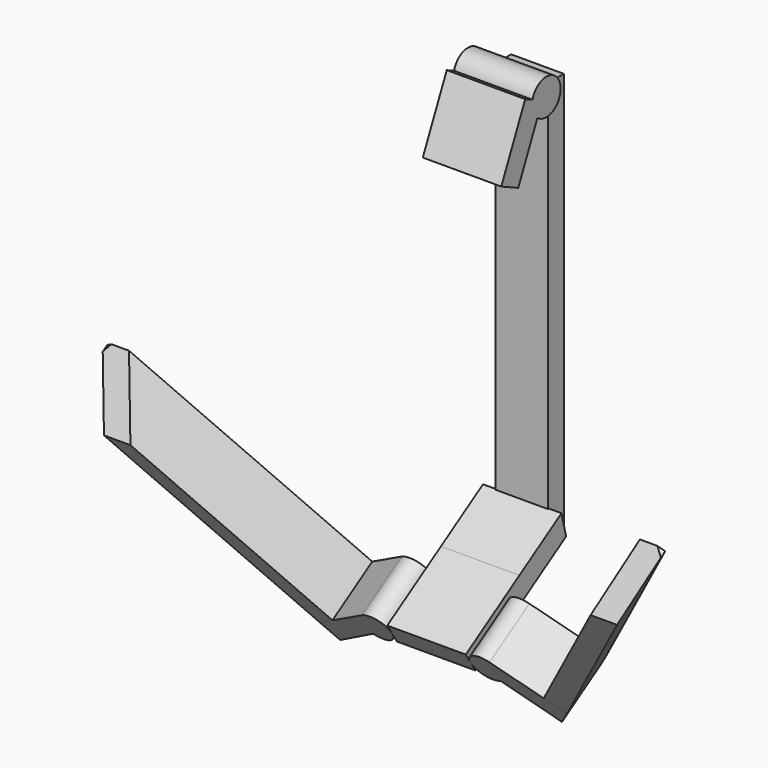
from build123d import *

# Parameters (mm, degrees)
F0_W           = 34.1221652925
F0_H           = 261.6441845894
F1_DEPTH       = 12.7
F3_DEPTH       = 25.4
F3_DEPTH_BACK  = 25.4
F7_DEPTH       = 25.4
F7_DEPTH_BACK  = 25.4
F9_DEPTH       = 38.1
F11_W          = 14.1206162959
F11_H          = 38.1
F12_DEPTH      = 177.8
F15_DEPTH      = 508
F15_DEPTH_BACK = 508
F20_DEPTH      = 228.6
F20_DEPTH_BACK = 228.6


with BuildPart() as f1:
    # F0 (on Front) → F1 (new body)
    with BuildSketch(Plane.XZ):
        Rectangle(F0_W, F0_H)
    extrude(amount=F1_DEPTH)


with BuildPart() as f3:
    # F2 (on Right) → F3 (new body, two sides)
    with BuildSketch(Plane.YZ) as f3_sk:
        with BuildLine():
            ThreePointArc((-31.7653294782, 121.3009119591), (-19.5443195923, 119.9093799667), (-12.9962554201, 130.3215026855))
            ThreePointArc((-12.9962554201, 130.3215026855), (-23.058684097, 141.777262991), (-35.7164542609, 133.2762177888))
            ThreePointArc((-35.7164542609, 133.2762177888), (-35.5190055596, 126.7018951749), (-31.7653294782, 121.3009119591))
        make_face()
        with BuildLine():
            ThreePointArc((-31.7653294782, 121.3009119591), (-35.5190055596, 126.7018951749), (-35.7164542609, 133.2762177888))
            Line((-35.7164542609, 133.2762177888), (-41.654221951, 136.0218451646))
            Line((-41.654221951, 136.0218451646), (-61.046799285, 94.0829352683))
            Line((-61.046799285, 94.0829352683), (-47.2919270396, 87.7226740122))
            Line((-47.2919270396, 87.7226740122), (-31.7653294782, 121.3009119591))
        make_face()
    extrude(amount=F3_DEPTH)
    extrude(f3_sk.sketch, amount=-F3_DEPTH_BACK)


with BuildPart() as f4_1:
    # F4: instance of F3
    add(f3.part.mirror(Plane.XY))


with BuildPart() as f7:
    # F6 (on Right) → F7 (new body, two sides)
    with BuildSketch(Plane.YZ) as f7_sk:
        Polygon((-82.0237547159, -173.1977909803), (-37.7950449612, -145.1887713173), (-8.5108920135, -126.643794078), (-12.3146369824, -111.9083875607), (-46.3577486399, -133.4671033607), (-89.7730322343, -160.9609990365), align=None)
    extrude(amount=F7_DEPTH)
    extrude(f7_sk.sketch, amount=-F7_DEPTH_BACK)


with BuildPart() as f9:
    # F8 (on face) → F9 (new body)
    with BuildSketch(Plane(origin=(0, -136.8311862758, -86.652027793), x_dir=(1, 0, 0), z_dir=(0, -0.8448406307, -0.5350180453))):
        with BuildLine():
            ThreePointArc((-41.2132547892, -103.603452681), (-30.7810506283, -104.152405518), (-25.4, -95.198270886))
            ThreePointArc((-25.4, -95.198270886), (-30.8167276914, -86.225263874), (-41.2799833491, -86.8385132228))
            ThreePointArc((-41.2799833491, -86.8385132228), (-45.680760801, -95.2386319206), (-41.2132547892, -103.603452681))
        make_face()
        with BuildLine():
            ThreePointArc((-41.2132547892, -103.603452681), (-45.680760801, -95.2386319206), (-41.2799833491, -86.8385132228))
            Line((-41.2799833491, -86.8385132228), (-80.0200754217, -113.4363166259))
            Line((-80.0200754217, -113.4363166259), (-71.7834234238, -125.1321434975))
            Line((-71.7834234238, -125.1321434975), (-41.2132547892, -103.603452681))
        make_face()
    extrude(amount=-F9_DEPTH)


with BuildPart() as f10_1:
    # F10: instance of F9
    add(f9.part.mirror(Plane.YZ))


with BuildPart() as f9_1:
    add(f9.part)

    # F11 (on face) → F12 (join)
    with BuildSketch(Plane(origin=(27.2956463477, 21.2704505823, -33.5879154814), x_dir=(0.8243995022, -0.302824685, 0.4781868578), z_dir=(-0.5660083575, -0.4410686102, 0.6964861954))):
        with Locations((-123.1141054526, -142.9109442375)):
            Rectangle(F11_W, F11_H)
    extrude(amount=F12_DEPTH)


with BuildPart() as f13_1:
    # F13: instance of F9
    add(f9_1.part.mirror(Plane.YZ))


with BuildPart() as f15_tool:
    # F14 (on Right) → F15 (new body, two sides)
    with BuildSketch(Plane.YZ) as f15_sk:
        Polygon((-170.909717679, -134.5487385988), (-87.3836744508, 40.231739617), (-170.909717679, 47.1544340253), align=None)
    extrude(amount=-F15_DEPTH)
    extrude(f15_sk.sketch, amount=F15_DEPTH_BACK)


with BuildPart() as f9_2:
    add(f9_1.part)

    # F15: cut by f15_tool
    add(f15_tool.part, mode=Mode.SUBTRACT)


with BuildPart() as f13_1_1:
    add(f13_1.part)

    # F15: cut by f15_tool
    add(f15_tool.part, mode=Mode.SUBTRACT)


with BuildPart() as f18_1:
    # F18: instance of F9
    add(f9_2.part.mirror(Plane.YZ))


with BuildPart() as f20:
    # F19 (on Right) → F20 (new body, two sides)
    with BuildSketch(Plane.YZ) as f20_sk:
        Polygon((-175.9073315984, -141.5651084215), (-144.9963003397, -76.4395818114), (-43.3924645185, 137.6264989376), (-107.6736316351, 168.8955078974), (-240.4824132121, -110.9153391191), align=None)
    extrude(amount=F20_DEPTH)
    extrude(f20_sk.sketch, amount=-F20_DEPTH_BACK)


solid = Compound([f1.part, f3.part, f7.part, f9_2.part, f18_1.part])
